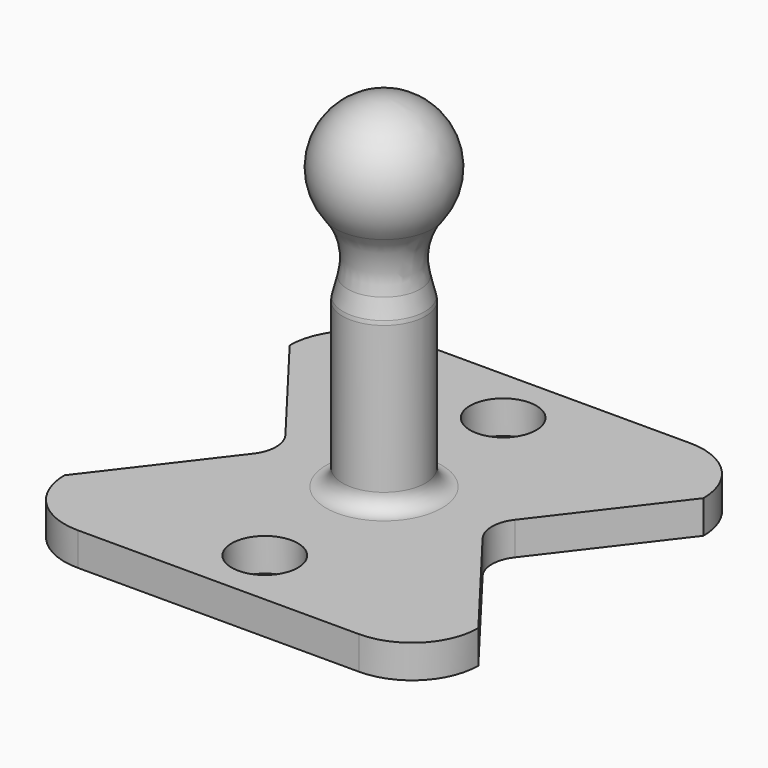
from build123d import *

# Parameters (mm, degrees)
F2_W     = 31.75
F2_H     = 31.75
F2_R     = 4.445
F3_DEPTH = 2.54
F4_R     = 5.08
F5_R     = 2.54
F6_DEPTH = 28.8935
F7_R     = 1.27
F9_DEPTH = 28.8935
F10_R    = 5.08


with BuildPart() as f1:
    # F0 (on Front) → F1 (revolve)
    with BuildSketch(Plane.XZ):
        with BuildLine():
            Line((0, 12.7), (0, 0))
            Line((0, 0), (3.175, 0))
            Line((3.175, 0), (4.445, 0))
            ThreePointArc((4.445, 0), (3.5469743879, 0.3719743879), (3.175, 1.27))
            Line((3.175, 1.27), (3.175, 12.7))
            Line((3.175, 12.7), (2.032, 17.2827523579))
            ThreePointArc((2.032, 17.2827523579), (4.6472934675, 22.6311866679), (0, 26.3525))
            Line((0, 26.3525), (0, 16.8275))
            Line((0, 16.8275), (0, 12.7))
        make_face()
    revolve(axis=Axis((0, 0, 21.59), (0, 0, 1)))

    # F7
    f7_edges = [f1.edges().sort_by_distance(p)[0] for p in [
        (-3.175, 0, 12.7),
    ]]
    fillet(f7_edges, radius=F7_R)

    # F10
    f10_edges = [f1.edges().sort_by_distance(p)[0] for p in [
        (-2.032, 0, 17.282752),
    ]]
    fillet(f10_edges, radius=F10_R)


with BuildPart() as f3:
    # F2 (on face) → F3 (new body)
    with BuildSketch(Plane(origin=(0, 0, 0), x_dir=(1, 0, 0), z_dir=(0, 0, -1))):
        Rectangle(F2_W, F2_H)
        Circle(F2_R, mode=Mode.SUBTRACT)
        Circle(F2_R)
    extrude(amount=F3_DEPTH)

    # F4
    f4_edges = [f3.edges().sort_by_distance(p)[0] for p in [
        (-15.875, -15.875, -1.27),
        (15.875, -15.875, -1.27),
        (15.875, 15.875, -1.27),
        (-15.875, 15.875, -1.27),
    ]]
    fillet(f4_edges, radius=F4_R)

    # F5 (on face) → F6 (cut, through all)
    with BuildSketch(Plane(origin=(0, 0, -2.54), x_dir=(1, 0, 0), z_dir=(0, 0, -1))):
        with Locations((0, 11.43)):
            Circle(F5_R)
        with Locations((0, -11.43)):
            Circle(F5_R)
    extrude(amount=-F6_DEPTH, mode=Mode.SUBTRACT)

    # F8 (on face) → F9 (cut, through all)
    with BuildSketch(Plane(origin=(0, 0, -2.54), x_dir=(1, 0, 0), z_dir=(0, 0, -1))):
        with BuildLine():
            Line((-8.7998825031, 1.5429232732), (-15.875, 10.795))
            Line((-15.875, 10.795), (-15.875, -10.795))
            Line((-15.875, -10.795), (-8.7998825031, -1.5429232732))
            ThreePointArc((-8.7998825031, -1.5429232732), (-8.2775513988, 0), (-8.7998825031, 1.5429232732))
        make_face()
        with BuildLine():
            Line((15.875, -10.795), (15.875, 10.795))
            Line((15.875, 10.795), (8.7998825031, 1.5429232732))
            ThreePointArc((8.7998825031, 1.5429232732), (8.2775513988, 0), (8.7998825031, -1.5429232732))
            Line((8.7998825031, -1.5429232732), (15.875, -10.795))
        make_face()
    extrude(amount=-F9_DEPTH, mode=Mode.SUBTRACT)


solid = Compound([f1.part, f3.part])
